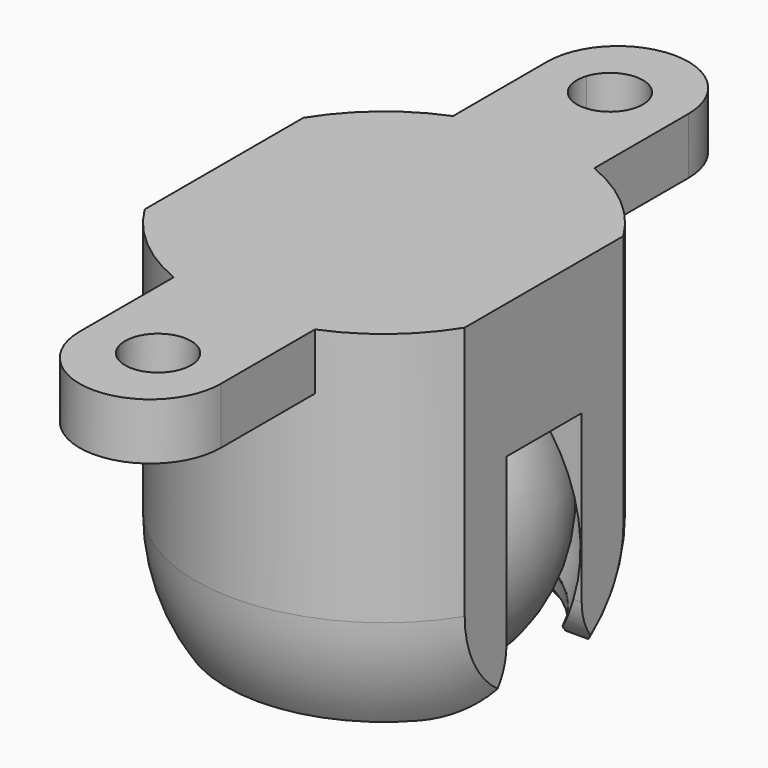
from build123d import *

# Parameters (mm, degrees)
F4_W         = 10.2586201175
F4_H         = 50.4137935346
F4_W_2       = 10.5517231097
F4_H_2       = 69.4655125564
F5_DEPTH     = 51.8
F6_W         = 5
F6_H         = 18
F7_DEPTH     = 12.5
F8_W         = 63.9707149493
F8_H         = 21.5102910659
F9_DEPTH     = 12.5
F10_T2_ANGLE = 177.2228091348
F10_T4_ANGLE = 177.2228091348
F12_DEPTH    = 3
F14_DEPTH    = 1
F15_T2_ANGLE = 159.9809066124
F15_T4_ANGLE = 159.9809066124
F16_T1_DEPTH = 15.5741640214
F16_T3_DEPTH = 15.5741640214
F17_R        = 0.1


# Not quite as in the source:
# - a fillet or chamfer that OpenCascade refuses, or shapes differently, is made with other operations: its cross-section is extruded or revolved along the edge and cut away or added


with BuildPart() as f1:
    # F0 (on Front) → F1 (revolve)
    with BuildSketch(Plane.XZ):
        with BuildLine():
            Line((0, -5), (0, -20.875))
            ThreePointArc((0, -20.875), (7.9375, -12.9375), (0, -5))
        make_face()
    revolve(axis=Axis((0, 0, -12.9375), (0, 0, 1)))


with BuildPart() as f3:
    # F2 (on Front) → F3 (revolve)
    with BuildSketch(Plane.XZ):
        with BuildLine():
            Line((-10, 0), (-10, -13.5))
            ThreePointArc((-10, -13.5), (-7.0710678119, -20.5710678119), (0, -23.5))
            Line((0, -23.5), (0, -22.3))
            ThreePointArc((0, -22.3), (-8.8, -13.5), (0, -4.7))
            Line((0, -4.7), (0, -3.5))
            Line((0, -3.5), (0, 0))
            Line((0, 0), (-10, 0))
        make_face()
    revolve(axis=Axis((0, 0, -11.75), (0, 0, -1)))

    # F4 (on Top) → F5 (cut)
    with BuildSketch(Plane.XY):
        with Locations((-13.6293100588, 1.746626564)):
            Rectangle(F4_W, F4_H)
        with Locations((13.7758615549, -0.1585464925)):
            Rectangle(F4_W_2, F4_H_2)
    extrude(amount=-F5_DEPTH, mode=Mode.SUBTRACT)

    # F6 (on Right) → F7 (cut, symmetric)
    with BuildSketch(Plane.YZ):
        with Locations((0, -16.1554028392)):
            Rectangle(F6_W, F6_H)
    extrude(amount=F7_DEPTH, both=True, mode=Mode.SUBTRACT)

    # F8 (on Front) → F9 (cut, symmetric)
    with BuildSketch(Plane.XZ):
        with Locations((4.1476953775, -29.755145533)):
            Rectangle(F8_W, F8_H)
    extrude(amount=F9_DEPTH, both=True, mode=Mode.SUBTRACT)

    # F10: chamfer of 1 on 2 edges, made by hand

    # F10_s1 → F10_t2 (revolve, cut)
    with BuildSketch(Plane(origin=(0, 0, 0), x_dir=(0, 0, 1), z_dir=(-0.0242331898, 0.9997063331, 0))):
        with BuildLine():
            Line((-19.0351099352, -7.8248676366), (-18.2246731237, -7.3824879962))
            Line((-18.2246731237, -7.3824879962), (-18.2138554349, -7.3656660579))
            ThreePointArc((-18.2138554349, -7.3656660579), (-18.6180707549, -7.1339856846), (-18.9875, -6.8538853032))
            Line((-18.9875, -6.8538853032), (-19.02, -6.8694977982))
            ThreePointArc((-19.02, -6.8694977982), (-19.02, -7.3471827174), (-19.0551099352, -7.8248676366))
            Line((-19.0551099352, -7.8248676366), (-19.0351099352, -7.8248676366))
        make_face()
    revolve(axis=Axis((0, 0, -19), (0, 0, 1)), revolution_arc=F10_T2_ANGLE, mode=Mode.SUBTRACT)

    # F10_s3 → F10_t4 (revolve, cut)
    with BuildSketch(Plane(origin=(0, 0, 0), x_dir=(0, 0, 1), z_dir=(0.0242331898, -0.9997063331, 0))):
        with BuildLine():
            Line((-19.0351099352, -7.8248676366), (-18.2246731237, -7.3824879962))
            Line((-18.2246731237, -7.3824879962), (-18.2138554349, -7.3656660579))
            ThreePointArc((-18.2138554349, -7.3656660579), (-18.6180707549, -7.1339856846), (-18.9875, -6.8538853032))
            Line((-18.9875, -6.8538853032), (-19.02, -6.8694977982))
            ThreePointArc((-19.02, -6.8694977982), (-19.02, -7.3471827174), (-19.0551099352, -7.8248676366))
            Line((-19.0551099352, -7.8248676366), (-19.0351099352, -7.8248676366))
        make_face()
    revolve(axis=Axis((0, 0, -19), (0, 0, 1)), revolution_arc=F10_T4_ANGLE, mode=Mode.SUBTRACT)

    # F11 (on Top) → F12 (join)
    with BuildSketch(Plane.XY):
        with BuildLine():
            Line((3.75, 9.2702481089), (3.75, 15.5202481089))
            Line((3.75, 15.5202481089), (1.6708805778, 15.5202481089))
            ThreePointArc((1.6708805778, 15.5202481089), (1.7301070792, 15.2631149833), (1.75, 15))
            ThreePointArc((1.75, 15), (-0.2631149833, 13.2698929208), (-1.6708805778, 15.5202481089))
            Line((-1.6708805778, 15.5202481089), (-3.75, 15.5202481089))
            Line((-3.75, 15.5202481089), (-3.75, 9.2702481089))
            Line((-3.75, 9.2702481089), (3.75, 9.2702481089))
        make_face()
        with BuildLine():
            Line((1.6708805778, 15.5202481089), (3.75, 15.5202481089))
            ThreePointArc((3.75, 15.5202481089), (0, 19.2702481089), (-3.75, 15.5202481089))
            Line((-3.75, 15.5202481089), (-1.6708805778, 15.5202481089))
            ThreePointArc((-1.6708805778, 15.5202481089), (0, 16.75), (1.6708805778, 15.5202481089))
        make_face()
        with BuildLine():
            Line((3.75, -9.2702481089), (-3.75, -9.2702481089))
            Line((-3.75, -9.2702481089), (-3.75, -15.5202481089))
            Line((-3.75, -15.5202481089), (-1.6708805778, -15.5202481089))
            ThreePointArc((-1.6708805778, -15.5202481089), (-0.2631149833, -13.2698929208), (1.75, -15))
            ThreePointArc((1.75, -15), (1.7301070792, -15.2631149833), (1.6708805778, -15.5202481089))
            Line((1.6708805778, -15.5202481089), (3.75, -15.5202481089))
            Line((3.75, -15.5202481089), (3.75, -9.2702481089))
        make_face()
        with BuildLine():
            Line((-1.6708805778, -15.5202481089), (-3.75, -15.5202481089))
            ThreePointArc((-3.75, -15.5202481089), (0, -19.2702481089), (3.75, -15.5202481089))
            Line((3.75, -15.5202481089), (1.6708805778, -15.5202481089))
            ThreePointArc((1.6708805778, -15.5202481089), (0, -16.75), (-1.6708805778, -15.5202481089))
        make_face()
    extrude(amount=-F12_DEPTH)

    # F13 (on face) → F14 (cut)
    with BuildSketch(Plane(origin=(0, 0, -3), x_dir=(1, 0, 0), z_dir=(0, 0, -1))):
        Polygon((-3, -16.7320508076), (0, -18.4641016151), (3, -16.7320508076), (3, -13.2679491924), (0, -11.5358983849), (-3, -13.2679491924), align=None)
        Polygon((-3, 13.2679491924), (0, 11.5358983849), (3, 13.2679491924), (3, 16.7320508076), (0, 18.4641016151), (-3, 16.7320508076), align=None)
    extrude(amount=-F14_DEPTH, mode=Mode.SUBTRACT)

    # F15: chamfer of 0.5 on 2 edges, made by hand

    # F15_s1 → F15_t2 (revolve, cut)
    with BuildSketch(Plane(origin=(0, 0, 0), x_dir=(0, 0, 1), z_dir=(0.1738122651, 0.9847788059, 0))):
        with BuildLine():
            Line((-17.8437964827, 7.6420038501), (-18.7053030152, 7.6337328607))
            Line((-18.7053030152, 7.6337328607), (-18.710094234, 7.6249553769))
            ThreePointArc((-18.710094234, 7.6249553769), (-18.4849984105, 7.5131946369), (-18.2645742778, 7.3928753878))
            Line((-18.2645742778, 7.3928753878), (-18.2543742145, 7.3932419024))
            ThreePointArc((-18.2543742145, 7.3932419024), (-18.0508300427, 7.5202424111), (-17.8388376241, 7.633319973))
            Line((-17.8388376241, 7.633319973), (-17.8437964827, 7.6420038501))
        make_face()
    revolve(axis=Axis((0, 0, -18.2597830589), (0, 0, -1)), revolution_arc=F15_T2_ANGLE, mode=Mode.SUBTRACT)

    # F15_s3 → F15_t4 (revolve, cut)
    with BuildSketch(Plane(origin=(0, 0, 0), x_dir=(0, 0, 1), z_dir=(-0.1738122651, -0.9847788059, 0))):
        with BuildLine():
            Line((-18.7053030152, 7.6337328607), (-17.8437964827, 7.6420038501))
            Line((-17.8437964827, 7.6420038501), (-17.8388376241, 7.633319973))
            ThreePointArc((-17.8388376241, 7.633319973), (-18.0508300427, 7.5202424111), (-18.2543742145, 7.3932419024))
            Line((-18.2543742145, 7.3932419024), (-18.2645742778, 7.3928753878))
            ThreePointArc((-18.2645742778, 7.3928753878), (-18.4849984105, 7.5131946369), (-18.710094234, 7.6249553769))
            Line((-18.710094234, 7.6249553769), (-18.7053030152, 7.6337328607))
        make_face()
    revolve(axis=Axis((0, 0, -18.2597830589), (0, 0, -1)), revolution_arc=F15_T4_ANGLE, mode=Mode.SUBTRACT)

    # F16: fillet of radius 3 on 4 edges, made by hand

    # F16_s2 → F16_t1 (cut)
    with BuildSketch(Plane.YZ.offset(-0.1054752961)):
        with BuildLine():
            ThreePointArc((-2.5, -16), (-3.3786796564, -18.1213203436), (-5.5, -19))
            Line((-5.5, -19), (-2.5, -19))
            Line((-2.5, -19), (-2.5, -16))
        make_face()
        with BuildLine():
            ThreePointArc((2.5, -16), (3.3786796564, -18.1213203436), (5.5, -19))
            Line((5.5, -19), (2.5, -19))
            Line((2.5, -19), (2.5, -16))
        make_face()
    extrude(amount=F16_T1_DEPTH, mode=Mode.SUBTRACT)

    # F16_s4 → F16_t3 (cut)
    with BuildSketch(Plane.YZ.offset(-15.4686887253)):
        with BuildLine():
            ThreePointArc((-2.5, -16), (-3.3786796564, -18.1213203436), (-5.5, -19))
            Line((-5.5, -19), (-2.5, -19))
            Line((-2.5, -19), (-2.5, -16))
        make_face()
        with BuildLine():
            ThreePointArc((2.5, -16), (3.3786796564, -18.1213203436), (5.5, -19))
            Line((5.5, -19), (2.5, -19))
            Line((2.5, -19), (2.5, -16))
        make_face()
    extrude(amount=F16_T3_DEPTH, mode=Mode.SUBTRACT)

    # F17
    f17_edges = [f3.edges().sort_by_distance(p)[0] for p in [
        (0, -7.641812, -17.863796),
        (0, 7.641812, -17.863796),
    ]]
    fillet(f17_edges, radius=F17_R)


solid = Compound([f1.part, f3.part])
